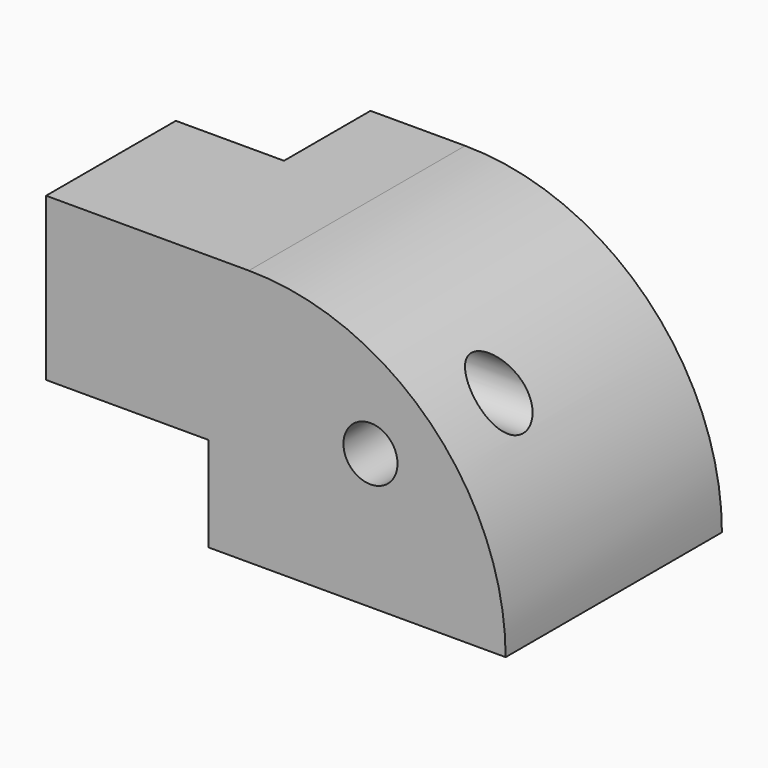
from build123d import *

# Parameters (mm, degrees)
F0_W     = 127
F0_H     = 120.65
F1_DEPTH = 215.9
F2_W     = 76.2
F2_H     = 44.45
F3_DEPTH = 127
F4_W     = 50.8
F4_H     = 76.2
F5_DEPTH = 50.8
F8_D     = 25.4
F8_DEPTH = 127
F8_TIP   = 7.6309298617
F9_R     = 120.64999
F10_D    = 25.4


# Not quite as in the source:
# - a fillet or chamfer is up to 0.001 mm smaller than in the source, because OpenCascade refuses the exact size


with BuildPart() as f1:
    # F0 (on Right) → F1 (new body)
    with BuildSketch(Plane.YZ):
        Rectangle(F0_W, F0_H)
    extrude(amount=F1_DEPTH)

    # F2 (on face) → F3 (cut)
    with BuildSketch(Plane.XZ.offset(63.5)):
        with Locations((38.1, -38.1)):
            Rectangle(F2_W, F2_H)
    extrude(amount=-F3_DEPTH, mode=Mode.SUBTRACT)

    # F4 (on face) → F5 (cut)
    with BuildSketch(Plane(origin=(0, 0, 0), x_dir=(0, -1, 0), z_dir=(-1, 0, 0))):
        with Locations((-38.1, 22.225)):
            Rectangle(F4_W, F4_H)
    extrude(amount=-F5_DEPTH, mode=Mode.SUBTRACT)

    # F8
    with Locations(Plane.XZ.offset(63.5)):
        with Locations((152.4, 3.175)):
            Hole(F8_D / 2, depth=F8_DEPTH)
            with Locations((0, 0, -(F8_DEPTH + F8_TIP / 2))):  # 118° drill point
                Cone(0, F8_D / 2, F8_TIP, mode=Mode.SUBTRACT)

    # F9 (radius 120.65 in the source; OpenCascade refuses exactly that, so slightly less here)
    f9_edges = [f1.edges().sort_by_distance(p)[0] for p in [
        (215.9, 0, 60.325),
    ]]
    fillet(f9_edges, radius=F9_R)

    # F10 (through all)
    with Locations(Plane(origin=(0, 0, 0), x_dir=(0, -1, 0), z_dir=(-1, 0, 0))):
        with Locations((25.4, 22.225)):
            Hole(F10_D / 2)


solid = f1.part
